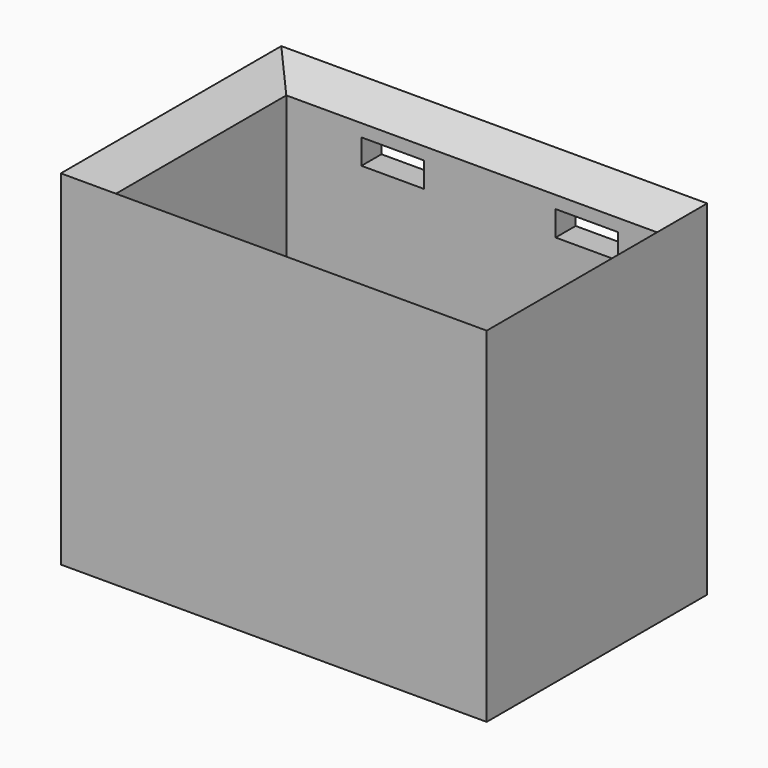
from build123d import *

# Parameters (mm, degrees)
F0_W         = 34
F0_H         = 22
F1_DEPTH     = 3
F2_W         = 34
F2_H         = 22
F2_W_2       = 30
F2_H_2       = 18
F3_DEPTH     = 24.5
F4_SIZE      = 1.99999
F5_W         = 5
F5_H         = 2
F6_DEPTH     = 2
F7_TEXT_SIZE = 6.6313349331
F8_DEPTH     = 1


# Not quite as in the source:
# - a fillet or chamfer is up to 0.001 mm smaller than in the source, because OpenCascade refuses the exact size
# - Text() gives the source's letters only with a copy of the font that has no kerning and outlines rounded to 1/6400 em; it was checked with that copy


with BuildPart() as f1:
    # F0 (on Top) → F1 (new body)
    with BuildSketch(Plane.XY):
        Rectangle(F0_W, F0_H)
    extrude(amount=F1_DEPTH)

    # F2 (on face) → F3 (join)
    with BuildSketch(Plane.XY.offset(3)):
        Rectangle(F2_W, F2_H)
        Rectangle(F2_W_2, F2_H_2, mode=Mode.SUBTRACT)
    extrude(amount=F3_DEPTH)

    # F4 (size 2 in the source; OpenCascade refuses exactly that, so slightly less here)
    f4_edges = [f1.edges().sort_by_distance(p)[0] for p in [
        (-15, 0, 27.5),
        (15, 0, 27.5),
        (0, -9, 27.5),
        (0, 9, 27.5),
    ]]
    chamfer(f4_edges, length=F4_SIZE)

    # F5 (on face) → F6 (cut)
    with BuildSketch(Plane(origin=(0, 11, 0), x_dir=(-1, 0, 0), z_dir=(0, 1, 0))):
        with Locations((-9, 23.5)):
            Rectangle(F5_W, F5_H)
        with Locations((6.5, 23.5)):
            Rectangle(F5_W, F5_H)
    extrude(amount=-F6_DEPTH, mode=Mode.SUBTRACT)

    # F7 (on face) → F8 (join)
    with BuildSketch(Plane(origin=(0, 11, 0), x_dir=(-1, 0, 0), z_dir=(0, 1, 0))):
        with Locations((-11.4098209888, 9.0557215735)):
            Text('SOLAR', F7_TEXT_SIZE, font='Open Sans', font_style=FontStyle.BOLD, text_align=(TextAlign.LEFT, TextAlign.BOTTOM))
    extrude(amount=F8_DEPTH)


solid = f1.part
